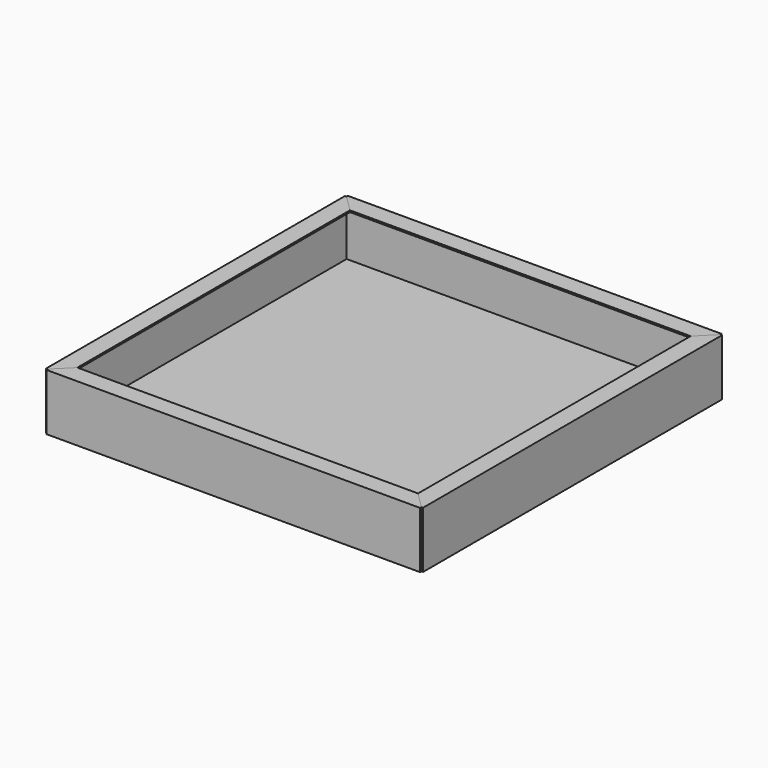
from build123d import *

# Parameters (mm, degrees)
F0_W     = 340
F0_H     = 340
F1_DEPTH = 1.5
F2_W     = 340
F2_H     = 50
F3_DEPTH = 1.5
F5_COUNT = 4
F7_DEPTH = 1.5
F8_COUNT = 4


with BuildPart() as f1:
    # F0 (on Top) → F1 (new body)
    with BuildSketch(Plane.XY):
        Rectangle(F0_W, F0_H)
    extrude(amount=F1_DEPTH)


with BuildPart() as f3:
    # F2 (on face) → F3 (new body)
    with BuildSketch(Plane.XZ.offset(170)):
        with Locations((0, 25)):
            Rectangle(F2_W, F2_H)
    extrude(amount=F3_DEPTH)


with BuildPart() as f5_1:
    # F5: instance of F3
    add(f3.part.rotate(Axis((0, 0, 1.5), (0, 0, 1)), 1 * 360 / F5_COUNT))


with BuildPart() as f5_2:
    # F5: instance of F3
    add(f3.part.rotate(Axis((0, 0, 1.5), (0, 0, 1)), 2 * 360 / F5_COUNT))


with BuildPart() as f5_3:
    # F5: instance of F3
    add(f3.part.rotate(Axis((0, 0, 1.5), (0, 0, 1)), 3 * 360 / F5_COUNT))


with BuildPart() as f3_1:
    add(f3.part)

    # F6 (on face) → F7 (join)
    with BuildSketch(Plane.XY.offset(50)):
        Polygon((-170, -170), (-170, -171.5), (170, -171.5), (170, -170), (155, -155), (-155, -155), align=None)
    extrude(amount=F7_DEPTH)


with BuildPart() as f8_1:
    # F8: instance of F3
    add(f3_1.part.rotate(Axis((0, 0, 1.5), (0, 0, 1)), 1 * 360 / F8_COUNT))


with BuildPart() as f8_2:
    # F8: instance of F3
    add(f3_1.part.rotate(Axis((0, 0, 1.5), (0, 0, 1)), 2 * 360 / F8_COUNT))


with BuildPart() as f8_3:
    # F8: instance of F3
    add(f3_1.part.rotate(Axis((0, 0, 1.5), (0, 0, 1)), 3 * 360 / F8_COUNT))


solid = Compound([f1.part, f5_1.part, f5_2.part, f5_3.part, f3_1.part, f8_1.part, f8_2.part, f8_3.part])
